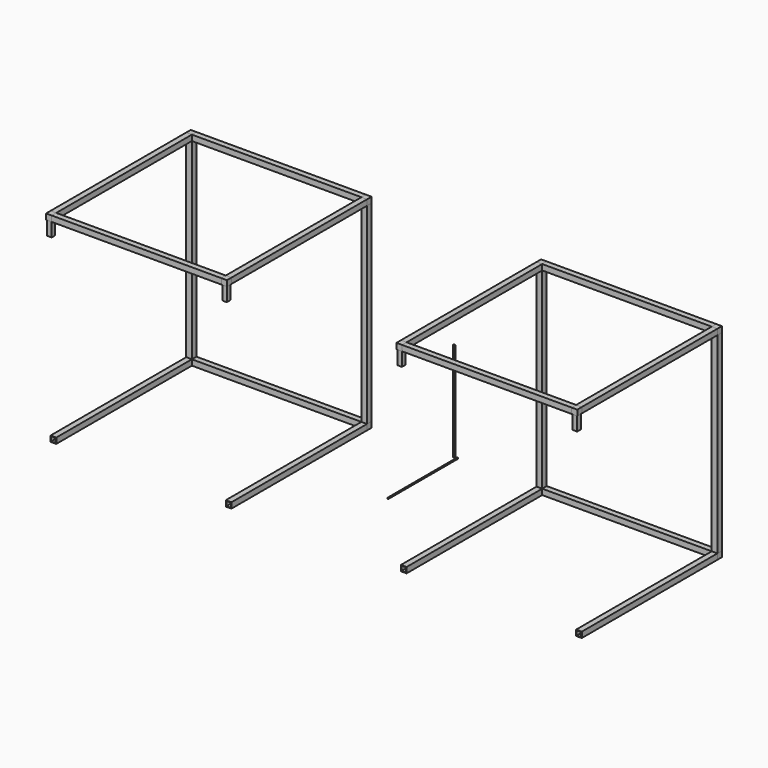
from build123d import *

# Parameters (mm, degrees)
F0_W      = 20
F0_H      = 20
F1_DEPTH  = 10
F2_W      = 16
F2_H      = 16
F8_DEPTH  = 50
F5_W      = 16
F5_H      = 16
F3_W      = 16
F3_H      = 16
F9_DEPTH  = 50
F4_W      = 16
F4_H      = 16
F10_DEPTH = 50
F7_W      = 16
F7_H      = 16
F6_W      = 16
F6_H      = 16
F11_DEPTH = 50
F12_DEPTH = 600
F13_DEPTH = 600
F14_W     = 4.7080824152
F14_H     = 4.7398181632
F15_DEPTH = 350
F16_DEPTH = 680
F19_W     = 2.552789636
F19_H     = 3.5656793043
F20_DEPTH = 310


# Not quite as in the source:
# - a feature names something its author has since deleted; it is built from what else it names


with BuildPart() as f1:
    # F0 (on Front) → F1 (new body, symmetric)
    with BuildSketch(Plane.XZ):
        with Locations((310, 0)):
            Rectangle(F0_W, F0_H)
    extrude(amount=F1_DEPTH, both=True)

    # F2 (on face) → F8 (join)
    with BuildSketch(Plane.XZ.offset(10)):
        with Locations((310, 0)):
            Rectangle(F2_W, F2_H)
    extrude(amount=F8_DEPTH)

    # F3 (on face) → F9 (join)
    with BuildSketch(Plane.YZ.offset(320)):
        Rectangle(F3_W, F3_H)
    extrude(amount=F9_DEPTH)

    # F4 (on face) → F10 (join)
    with BuildSketch(Plane.XY.offset(10)):
        with Locations((310, 0)):
            Rectangle(F4_W, F4_H)
    extrude(amount=F10_DEPTH)


with BuildPart() as f1b:
    # F0 (on Front) → F1, piece 2 (new body, symmetric)
    with BuildSketch(Plane.XZ):
        with Locations((930, 0)):
            Rectangle(F0_W, F0_H)
    extrude(amount=F1_DEPTH, both=True)

    # F5 (on face) → F8, piece 2 (join)
    with BuildSketch(Plane.XZ.offset(10)):
        with Locations((930, 0)):
            Rectangle(F5_W, F5_H)
    extrude(amount=F8_DEPTH)

    # F7 (on face) → F10, piece 2 (join)
    with BuildSketch(Plane.XY.offset(10)):
        with Locations((930, 0)):
            Rectangle(F7_W, F7_H)
    extrude(amount=F10_DEPTH)

    # F6 (on face) → F11 (join)
    with BuildSketch(Plane(origin=(920, 0, 0), x_dir=(0, -1, 0), z_dir=(-1, 0, 0))):
        Rectangle(F6_W, F6_H)
    extrude(amount=F11_DEPTH)


with BuildPart() as f12:
    # F12 (new, through all): a face of the model
    f12_faces = [f1.part.faces().sort_by_distance(p)[0] for p in [
        (320, 9.7171572875, 0),
    ]]
    extrude(f12_faces, amount=F12_DEPTH)


with BuildPart() as f13:
    # F13 (new): a face of the model
    f13_faces = [f1.part.faces().sort_by_distance(p)[0] for p in [
        (310, -10, 9.7171572875),
    ]]
    extrude(f13_faces, amount=F13_DEPTH)


with BuildPart() as f13b:
    # F13#2 (new): a face of the model
    f13_2_faces = [f1b.part.faces().sort_by_distance(p)[0] for p in [
        (930, -10, 9.7171572875),
    ]]
    extrude(f13_2_faces, amount=F13_DEPTH)


with BuildPart() as f15:
    # F14 (on Top) → F15 (new body)
    with BuildSketch(Plane.XY):
        Rectangle(F14_W, F14_H)
    extrude(amount=F15_DEPTH)


with BuildPart() as f16:
    # F16 (new): a face of the model
    f16_faces = [f1.part.faces().sort_by_distance(p)[0] for p in [
        (310, 9.7171572875, 10),
    ]]
    extrude(f16_faces, amount=F16_DEPTH)


with BuildPart() as f16b:
    # F16#2 (new): a face of the model
    f16_2_faces = [f1b.part.faces().sort_by_distance(p)[0] for p in [
        (930, 9.7171572875, 10),
    ]]
    extrude(f16_2_faces, amount=F16_DEPTH)


with BuildPart() as f17_1:
    # F17: instance of F13
    add(f13.part.mirror(Plane.XY.offset(350)))


with BuildPart() as f17_2:
    # F17: instance of F13b
    add(f13b.part.mirror(Plane.XY.offset(350)))


with BuildPart() as f17_3:
    # F17: instance of F1
    add(f1.part.mirror(Plane.XY.offset(350)))


with BuildPart() as f17_4:
    # F17: instance of F12
    add(f12.part.mirror(Plane.XY.offset(350)))


with BuildPart() as f17_5:
    # F17: instance of F1b
    add(f1b.part.mirror(Plane.XY.offset(350)))


with BuildPart() as f18_1:
    # F18: instance of F1b
    add(f1b.part.mirror(Plane.YZ))


with BuildPart() as f18_2:
    # F18: instance of F17_5
    add(f17_5.part.mirror(Plane.YZ))


with BuildPart() as f18_3:
    # F18: instance of F17_1
    add(f17_1.part.mirror(Plane.YZ))


with BuildPart() as f18_4:
    # F18: instance of F17_2
    add(f17_2.part.mirror(Plane.YZ))


with BuildPart() as f18_5:
    # F18: instance of F17_3
    add(f17_3.part.mirror(Plane.YZ))


with BuildPart() as f18_6:
    # F18: instance of F17_4
    add(f17_4.part.mirror(Plane.YZ))


with BuildPart() as f18_7:
    # F18: instance of F16
    add(f16.part.mirror(Plane.YZ))


with BuildPart() as f18_8:
    # F18: instance of F16b
    add(f16b.part.mirror(Plane.YZ))


with BuildPart() as f18_9:
    # F18: instance of F12
    add(f12.part.mirror(Plane.YZ))


with BuildPart() as f18_10:
    # F18: instance of F13
    add(f13.part.mirror(Plane.YZ))


with BuildPart() as f18_11:
    # F18: instance of F13b
    add(f13b.part.mirror(Plane.YZ))


with BuildPart() as f18_12:
    # F18: instance of F1
    add(f1.part.mirror(Plane.YZ))


with BuildPart() as f20:
    # F19 (on Front) → F20 (new body)
    with BuildSketch(Plane.XZ):
        with Locations((13.3685986511, 1.7828396522)):
            Rectangle(F19_W, F19_H)
    extrude(amount=F20_DEPTH)


with BuildPart() as f21_1:
    # F21: instance of F17_4
    add(f17_4.part.mirror(Plane(origin=(13.3685986511, -310, 1.7828396522), x_dir=(1, 0, 0), z_dir=(0, -1, 0))))


with BuildPart() as f21_2:
    # F21: instance of F17_3
    add(f17_3.part.mirror(Plane(origin=(13.3685986511, -310, 1.7828396522), x_dir=(1, 0, 0), z_dir=(0, -1, 0))))


with BuildPart() as f21_3:
    # F21: instance of F17_5
    add(f17_5.part.mirror(Plane(origin=(13.3685986511, -310, 1.7828396522), x_dir=(1, 0, 0), z_dir=(0, -1, 0))))


with BuildPart() as f21_4:
    # F21: instance of F18_6
    add(f18_6.part.mirror(Plane(origin=(13.3685986511, -310, 1.7828396522), x_dir=(1, 0, 0), z_dir=(0, -1, 0))))


with BuildPart() as f21_5:
    # F21: instance of F18_5
    add(f18_5.part.mirror(Plane(origin=(13.3685986511, -310, 1.7828396522), x_dir=(1, 0, 0), z_dir=(0, -1, 0))))


with BuildPart() as f21_6:
    # F21: instance of F18_2
    add(f18_2.part.mirror(Plane(origin=(13.3685986511, -310, 1.7828396522), x_dir=(1, 0, 0), z_dir=(0, -1, 0))))


solid = Compound([f1.part, f1b.part, f12.part, f13.part, f13b.part, f15.part, f16.part, f16b.part, f17_1.part, f17_2.part, f17_3.part, f17_4.part, f17_5.part, f18_1.part, f18_2.part, f18_3.part, f18_4.part, f18_5.part, f18_6.part, f18_7.part, f18_8.part, f18_9.part, f18_10.part, f18_11.part, f18_12.part, f20.part, f21_1.part, f21_2.part, f21_3.part, f21_4.part, f21_5.part, f21_6.part])
